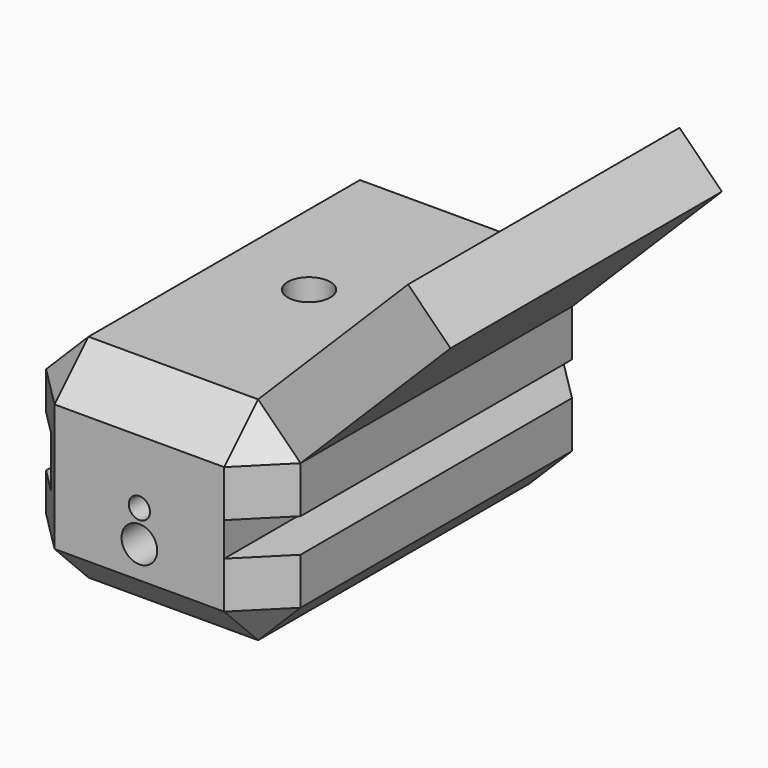
from build123d import *

# Parameters (mm, degrees)
F0_W     = 30
F0_H     = 50
F0_R     = 2.5
F1_DEPTH = 25
F2_SIZE  = 5
F4_DEPTH = 63.1
F6_DEPTH = 3
F8_D     = 4.2
F8_DEPTH = 20
F8_TIP   = 1.2618073
F9_DEPTH = 25
F11_D    = 2.5


with BuildPart() as f1:
    # F0 (on Top) → F1 (new body)
    with BuildSketch(Plane.XY):
        with Locations((15, 25)):
            Rectangle(F0_W, F0_H)
        with Locations((15, 25)):
            Circle(F0_R, mode=Mode.SUBTRACT)
    extrude(amount=F1_DEPTH)

    # F2
    f2_edges = [f1.edges().sort_by_distance(p)[0] for p in [
        (15, 50, 25),
        (30, 25, 25),
        (15, 0, 25),
        (0, 25, 25),
        (30, 25, 0),
        (15, 50, 0),
        (0, 25, 0),
        (15, 0, 0),
        (0, 0, 12.5),
        (30, 0, 12.5),
        (30, 50, 12.5),
        (0, 50, 12.5),
    ]]
    chamfer(f2_edges, length=F2_SIZE)

    # F3 (on face) → F4 (cut)
    with BuildSketch(Plane.XZ):
        Polygon((25, 14.5), (25, 12.5), (25, 10.5), (32.3230884969, 10.5), (32.3230884969, 14.5), align=None)
    extrude(amount=-F4_DEPTH, mode=Mode.SUBTRACT)

    # F5 (on face) → F6 (cut)
    with BuildSketch(Plane(origin=(0, 0, 0), x_dir=(0, -1, 0), z_dir=(-1, 0, 0))):
        with BuildLine():
            Line((-5, 15.5206739136), (-25.003100845, 15.4999983975))
            ThreePointArc((-25.003100845, 15.4999983975), (-27.9999995994, 12.4984495773), (-25, 9.5))
            Line((-25, 9.5), (-5, 9.5))
            Line((-5, 9.5), (-5, 15.5206739136))
        make_face()
        Polygon((7.2839763969, 15.5333708226), (-5, 15.5206739136), (-5, 9.5), (7.2839763969, 9.5), align=None)
    extrude(amount=-F6_DEPTH, mode=Mode.SUBTRACT)

    # F8
    with Locations(Plane.XZ):
        with Locations((15, 8.75)):
            Hole(F8_D / 2, depth=F8_DEPTH)
            with Locations((0, 0, -(F8_DEPTH + F8_TIP / 2))):  # 118° drill point
                Cone(0, F8_D / 2, F8_TIP, mode=Mode.SUBTRACT)


with BuildPart() as f9:
    # F9 (new): a face of the model
    f9_faces = [f1.part.faces().sort_by_distance(p)[0] for p in [
        (27.5, 25, 22.5),
    ]]
    extrude(f9_faces, amount=F9_DEPTH)


with BuildPart() as f1_1:
    add(f1.part)

    # F11 (through all)
    with Locations(Plane.XZ):
        with Locations((15, 12.5)):
            Hole(F11_D / 2)


solid = Compound([f9.part, f1_1.part])
